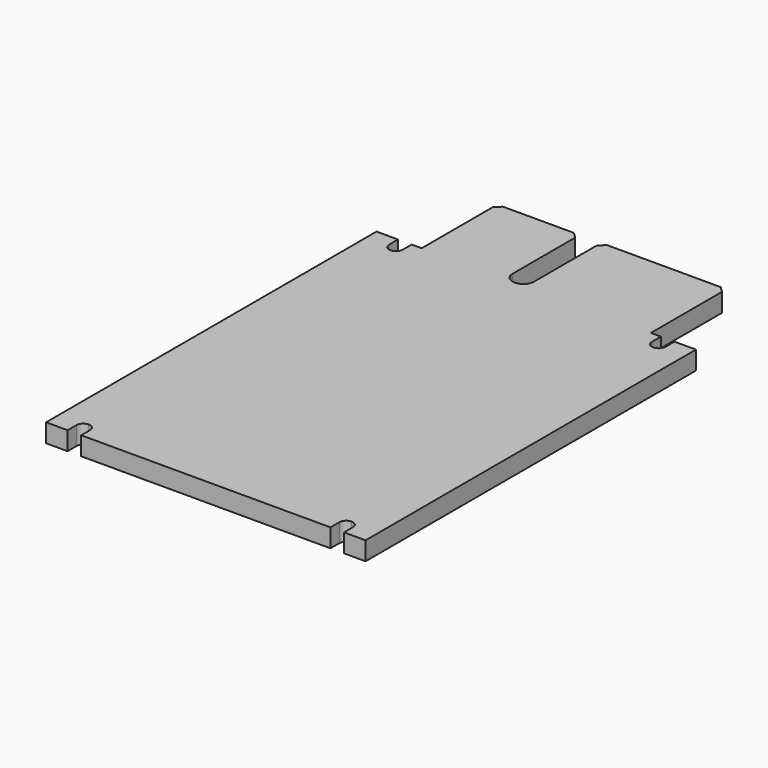
from build123d import *

# Parameters (mm, degrees)
F0_W     = 28.321
F0_H     = 45
F1_DEPTH = 1.64
F2_W     = 1.905
F2_H     = 8.382
F2_W_2   = 1.207
F2_H_2   = 1.5875
F3_DEPTH = 25
F4_R     = 0.95249
F5_SIZE  = 0.507
F6_R     = 0.60349


# Not quite as in the source:
# - a fillet or chamfer is up to 0.001 mm smaller than in the source, because OpenCascade refuses the exact size


with BuildPart() as f1:
    # F0 (on Top) → F1 (new body)
    with BuildSketch(Plane.XY):
        with Locations((0, -22.5)):
            Rectangle(F0_W, F0_H)
    extrude(amount=F1_DEPTH)

    # F2 (on Top) → F3 (cut)
    with BuildSketch(Plane.XY):
        Polygon((-10.1605, 0), (-14.1605, 0), (-14.1605, -8.382), (-12.2555, -8.382), (-12.2555, -9.9695), (-11.0485, -9.9695), (-11.0485, -8.382), (-10.1605, -8.382), align=None)
        with Locations((-1.905, -4.191)):
            Rectangle(F2_W, F2_H)
        Polygon((14.1605, -8.382), (14.1605, 0), (10.1595, 0), (10.1595, -8.382), (11.0485, -8.382), (11.0485, -9.9695), (12.2555, -9.9695), (12.2555, -8.382), align=None)
        with Locations((-11.652, -44.20625)):
            Rectangle(F2_W_2, F2_H_2)
        with Locations((11.652, -44.20625)):
            Rectangle(F2_W_2, F2_H_2)
    extrude(amount=F3_DEPTH, mode=Mode.SUBTRACT)

    # F4 (radius 0.9525 in the source; OpenCascade refuses exactly that, so slightly less here)
    f4_edges = [f1.edges().sort_by_distance(p)[0] for p in [
        (-2.8575, -8.382, 0.82),
        (-0.9525, -8.382, 0.82),
    ]]
    fillet(f4_edges, radius=F4_R)

    # F5
    f5_edges = [f1.edges().sort_by_distance(p)[0] for p in [
        (10.1595, 0, 0.82),
        (-0.9525, 0, 0.82),
        (-2.8575, 0, 0.82),
        (-10.1605, 0, 0.82),
    ]]
    chamfer(f5_edges, length=F5_SIZE)

    # F6 (radius 0.6035 in the source; OpenCascade refuses exactly that, so slightly less here)
    f6_edges = [f1.edges().sort_by_distance(p)[0] for p in [
        (12.2555, -43.4125, 0.82),
        (-12.2555, -43.4125, 0.82),
        (-11.0485, -43.4125, 0.82),
        (11.0485, -43.4125, 0.82),
        (11.0485, -9.9695, 0.82),
        (12.2555, -9.9695, 0.82),
        (-12.2555, -9.9695, 0.82),
        (-11.0485, -9.9695, 0.82),
    ]]
    fillet(f6_edges, radius=F6_R)


solid = f1.part
